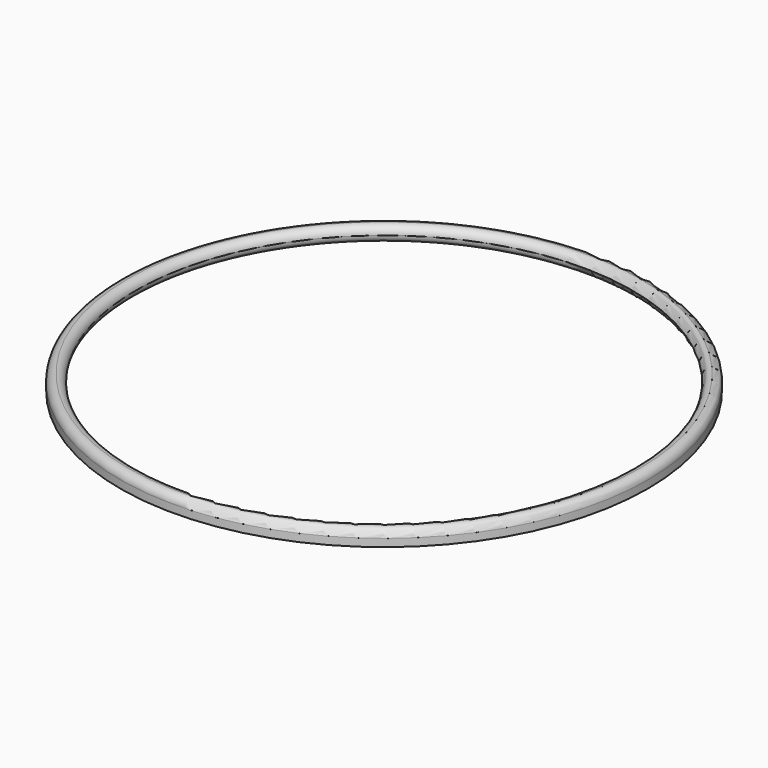
from build123d import *

# Parameters (mm, degrees)
F0_R     = 53.975
F0_R_2   = 50.8
F1_DEPTH = 3.175
F2_R     = 1.58749


# Not quite as in the source:
# - a fillet or chamfer is up to 0.001 mm smaller than in the source, because OpenCascade refuses the exact size


with BuildPart() as f1:
    # F0 (on Top) → F1 (new body)
    with BuildSketch(Plane.XY):
        Circle(F0_R)
        Circle(F0_R_2, mode=Mode.SUBTRACT)
    extrude(amount=F1_DEPTH)

    # F2 (radius 1.5875 in the source; OpenCascade refuses exactly that, so slightly less here)
    f2_edges = [f1.edges().sort_by_distance(p)[0] for p in [
        (-50.8, 0, 3.175),
        (-53.975, 0, 3.175),
        (-50.8, 0, 0),
    ]]
    fillet(f2_edges, radius=F2_R)


solid = f1.part
